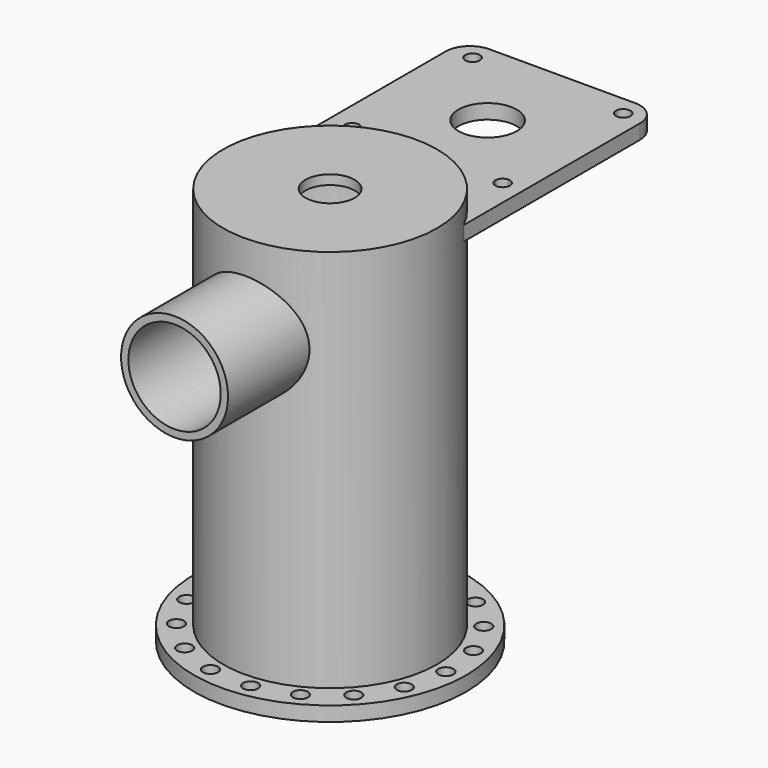
from build123d import *

# Parameters (mm, degrees)
F0_R            = 22
F1_DEPTH        = 82
F2_T            = -1.95
F0_R_2          = 28
F3_DEPTH        = 3
F5_R            = 5.05
F6_DEPTH        = 90
F7_R            = 1.55
F8_DEPTH        = 5
F8_COPIES_COUNT = 18
F10_R           = 11
F12_R           = 9.5
F13_DEPTH       = 30
F15_W           = 40
F15_H           = 3
F17_R           = 6
F18_DEPTH       = 10
F19_R           = 5


# Not quite as in the source:
# - a pattern or mirror of a feature is missing from the dataset's text; its kind, count and spacing are read off the source's solid


with BuildPart() as f1:
    # F0 (on Top) → F1 (new body)
    with BuildSketch(Plane.XY):
        Circle(F0_R)
    extrude(amount=F1_DEPTH)

    # F2
    f2_openings = [f1.faces().sort_by_distance(p)[0] for p in [
        (0, 0, 0),
    ]]
    offset(amount=F2_T, openings=f2_openings)

    # F0 (on Top) → F3 (join)
    with BuildSketch(Plane.XY):
        Circle(F0_R_2)
        Circle(F0_R, mode=Mode.SUBTRACT)
    extrude(amount=F3_DEPTH)

    # F5 (on Top) → F6 (cut)
    with BuildSketch(Plane.XY):
        Circle(F5_R)
    extrude(amount=F6_DEPTH, mode=Mode.SUBTRACT)

    # F7 (on face) → F8 (cut)
    with BuildSketch(Plane.XY):
        with Locations((-5.3322692402, -24.1057705134)):
            Circle(F7_R)
    f8 = extrude(amount=F8_DEPTH, mode=Mode.SUBTRACT)

    # F8_copies: F8 ×18 about axis
    f8_copies_axis = Axis((0, 0, 0), (0, 0, 1))
    for i in range(1, F8_COPIES_COUNT):
        add(f8.rotate(f8_copies_axis, i * 360 / F8_COPIES_COUNT), mode=Mode.SUBTRACT)

    # F10 (on offset) → F11 (join, up to the next surface of F1)
    with BuildSketch(Plane.XZ.offset(40)):
        with Locations((0, 64.2171450533)):
            Circle(F10_R)
    extrude(until=Until.NEXT, dir=(0, 1, 0))

    # F12 (on face) → F13 (cut)
    with BuildSketch(Plane.XZ.offset(40)):
        with Locations((0, 64.2171450533)):
            Circle(F12_R)
    extrude(amount=-F13_DEPTH, mode=Mode.SUBTRACT)

    # F15 (on offset) → F16 (join, up to the next surface of F1)
    with BuildSketch(Plane.XZ.offset(-60)):
        with Locations((-0.2395864576, 76.434844184)):
            Rectangle(F15_W, F15_H)
    extrude(until=Until.NEXT)

    # F17 (on face) → F18 (cut)
    with BuildSketch(Plane.XY.offset(82)):
        with BuildLine():
            Line((15.5, 56.001), (15.5, 54.501))
            ThreePointArc((15.5, 54.501), (16.5606601718, 54.9403398282), (17, 56.001))
            ThreePointArc((17, 56.001), (15.5, 57.501), (14, 56.001))
            Line((14, 56.001), (15.5, 56.001))
        make_face()
        with BuildLine():
            ThreePointArc((14, 56.001), (14.4393398282, 54.9403398282), (15.5, 54.501))
            Line((15.5, 54.501), (15.5, 56.001))
            Line((15.5, 56.001), (14, 56.001))
        make_face()
        with BuildLine():
            ThreePointArc((-14, 56.001), (-16.5606601718, 57.0616601718), (-15.5, 54.501))
            Line((-15.5, 54.501), (-15.5, 56.001))
            Line((-15.5, 56.001), (-14, 56.001))
        make_face()
        with BuildLine():
            Line((-15.5, 56.001), (-15.5, 54.501))
            ThreePointArc((-15.5, 54.501), (-14.4393398282, 54.9403398282), (-14, 56.001))
            Line((-14, 56.001), (-15.5, 56.001))
        make_face()
        with BuildLine():
            ThreePointArc((-15.5, 26.501), (-16.5606601718, 23.9403398282), (-14, 25.001))
            Line((-14, 25.001), (-15.5, 25.001))
            Line((-15.5, 25.001), (-15.5, 26.501))
        make_face()
        with BuildLine():
            Line((-15.5, 25.001), (-14, 25.001))
            ThreePointArc((-14, 25.001), (-14.4393398282, 26.0616601718), (-15.5, 26.501))
            Line((-15.5, 26.501), (-15.5, 25.001))
        make_face()
        with BuildLine():
            Line((15.5, 25.001), (14, 25.001))
            ThreePointArc((14, 25.001), (15.5, 23.501), (17, 25.001))
            ThreePointArc((17, 25.001), (16.5606601718, 26.0616601718), (15.5, 26.501))
            Line((15.5, 26.501), (15.5, 25.001))
        make_face()
        with BuildLine():
            ThreePointArc((15.5, 26.501), (14.4393398282, 26.0616601718), (14, 25.001))
            Line((14, 25.001), (15.5, 25.001))
            Line((15.5, 25.001), (15.5, 26.501))
        make_face()
        with Locations((0, 40.501)):
            Circle(F17_R)
    extrude(amount=-F18_DEPTH, mode=Mode.SUBTRACT)

    # F19
    f19_edges = [f1.edges().sort_by_distance(p)[0] for p in [
        (-20.239586, 60, 76.434844),
        (19.760414, 60, 76.434844),
    ]]
    fillet(f19_edges, radius=F19_R)


solid = f1.part
